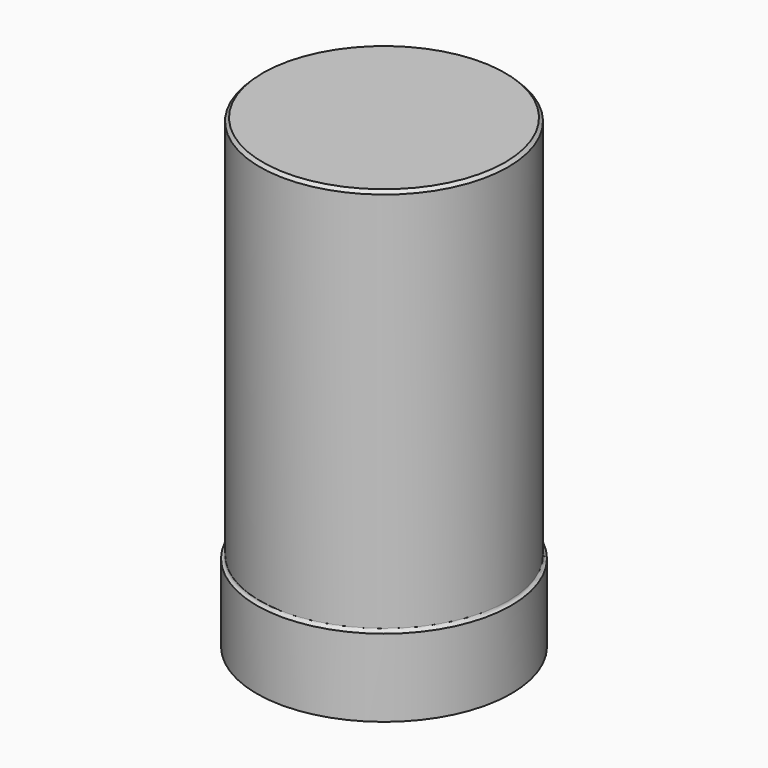
from build123d import *

# Parameters (mm, degrees)
F0_R     = 6
F1_DEPTH = 22.5
F2_R     = 6.15
F3_DEPTH = 3.75
F4_R     = 0.14999
F5_SIZE2 = 0.15
F5_SIZE  = 0.15


# Not quite as in the source:
# - a fillet or chamfer is up to 0.001 mm smaller than in the source, because OpenCascade refuses the exact size


with BuildPart() as f1:
    # F0 (on Top) → F1 (new body)
    with BuildSketch(Plane.XY):
        Circle(F0_R)
    extrude(amount=F1_DEPTH)

    # F2 (on Top) → F3 (join)
    with BuildSketch(Plane.XY):
        Circle(F2_R)
    extrude(amount=F3_DEPTH)

    # F4 (radius 0.15 in the source; OpenCascade refuses exactly that, so slightly less here)
    f4_edges = [f1.edges().sort_by_distance(p)[0] for p in [
        (-6, 0, 3.75),
    ]]
    fillet(f4_edges, radius=F4_R)

    # F5
    f5_edges = [f1.edges().sort_by_distance(p)[0] for p in [
        (-6, 0, 22.5),
    ]]
    chamfer(f5_edges, length=F5_SIZE, length2=F5_SIZE2)


solid = f1.part
